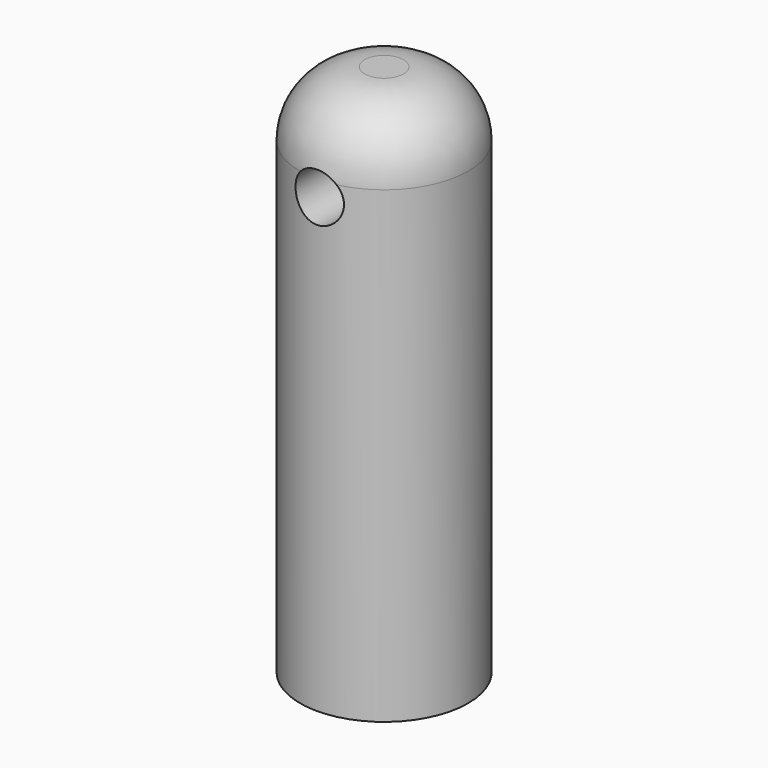
from build123d import *

# Parameters (mm, degrees)
F0_R      = 5.2
F0_R_2    = 2
F1_DEPTH  = 1.5
F2_R      = 5.2
F3_DEPTH  = 12.5
F4_R      = 5.2
F4_R_2    = 2
F5_DEPTH  = 13
F6_R      = 5.2
F7_DEPTH  = 6
F8_R      = 4
F9_R      = 1.5
F10_DEPTH = 12.5


with BuildPart() as f1:
    # F0 (on Top) → F1 (new body)
    with BuildSketch(Plane.XY):
        Circle(F0_R)
        Circle(F0_R_2, mode=Mode.SUBTRACT)
    extrude(amount=F1_DEPTH)

    # F2 (on face) → F3 (join)
    with BuildSketch(Plane.XY.offset(1.5)):
        Circle(F2_R)
        Polygon((0, 3.9259818305), (3.4, 1.9629909152), (3.4, -1.9629909152), (0, -3.9259818305), (-3.4, -1.9629909152), (-3.4, 1.9629909152), align=None, mode=Mode.SUBTRACT)
    extrude(amount=F3_DEPTH)

    # F4 (on face) → F5 (join)
    with BuildSketch(Plane.XY.offset(14)):
        Circle(F4_R)
        Polygon((-3.4, -1.9629909152), (-3.4, 1.9629909152), (0, 3.9259818305), (3.4, 1.9629909152), (3.4, -1.9629909152), (0, -3.9259818305), align=None, mode=Mode.SUBTRACT)
        Polygon((0, 3.9259818305), (-3.4, 1.9629909152), (-3.4, -1.9629909152), (0, -3.9259818305), (3.4, -1.9629909152), (3.4, 1.9629909152), align=None)
        Circle(F4_R_2, mode=Mode.SUBTRACT)
    extrude(amount=F5_DEPTH)

    # F6 (on face) → F7 (join)
    with BuildSketch(Plane.XY.offset(27)):
        Circle(F6_R)
    extrude(amount=F7_DEPTH)

    # F8
    f8_edges = [f1.edges().sort_by_distance(p)[0] for p in [
        (-5.2, 0, 33),
    ]]
    fillet(f8_edges, radius=F8_R)

    # F9 (on Front) → F10 (cut, symmetric)
    with BuildSketch(Plane.XZ):
        with Locations((0, 28)):
            Circle(F9_R)
    extrude(amount=F10_DEPTH, both=True, mode=Mode.SUBTRACT)


solid = f1.part
